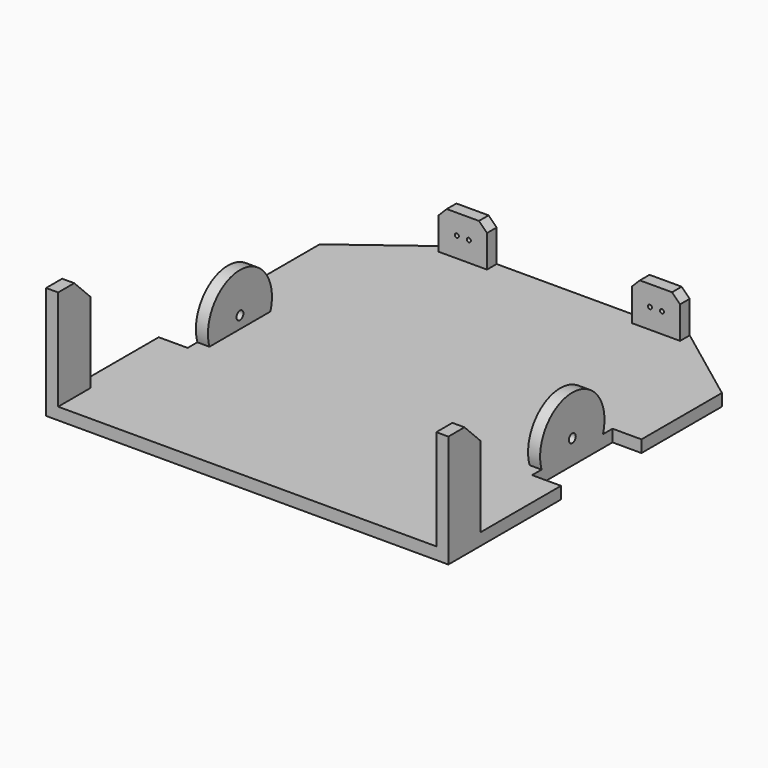
from build123d import *

# Parameters (mm, degrees)
F1_DEPTH  = 3
F2_R      = 1.075
F3_DEPTH  = 3
F4_R      = 1.075
F5_DEPTH  = 3
F6_W      = 12
F6_H      = 3
F7_DEPTH  = 10
F8_R      = 0.5
F9_DEPTH  = 3
F10_SIZE  = 2
F11_W     = 3
F11_H     = 10
F12_DEPTH = 25
F13_SIZE  = 5


# Not quite as in the source:
# - a feature names something its author has since deleted; it is built from what else it names


with BuildPart() as f1:
    # F0 (on Top) → F1 (new body)
    with BuildSketch(Plane.XY):
        Polygon((30, 56.1203770339), (-30, 56.1203770339), (-50, 41.1203770339), (-50, 16.1203770339), (-42.8093671799, 16.1203770339), (-42.8093671799, -8.8796229661), (-50, -8.8796229661), (-50, -43.8796229661), (50, -43.8796229661), (50, -8.8796229661), (42.8093671799, -8.8796229661), (42.8093671799, 16.1203770339), (50, 16.1203770339), (50, 41.1203770339), align=None)
    extrude(amount=F1_DEPTH)

    # F2 (on face) → F3 (join)
    with BuildSketch(Plane.YZ.offset(42.8093671799)):
        with BuildLine():
            Line((-5.9190149802, 3), (13.1597690481, 3))
            ThreePointArc((13.1597690481, 3), (3.6203770339, 16), (-5.9190149802, 3))
        make_face()
        with Locations((3.6203770339, 6)):
            Circle(F2_R, mode=Mode.SUBTRACT)
    extrude(amount=-F3_DEPTH)

    # F4 (on face) → F5 (join)
    with BuildSketch(Plane(origin=(-42.8093671799, 0, 0), x_dir=(0, -1, 0), z_dir=(-1, 0, 0))):
        with BuildLine():
            Line((-13.1019409746, 3), (5.8611869067, 3))
            ThreePointArc((5.8611869067, 3), (-3.6203770339, 15.9448506656), (-13.1019409746, 3))
        make_face()
        with Locations((-3.6203770339, 6)):
            Circle(F4_R, mode=Mode.SUBTRACT)
    extrude(amount=-F5_DEPTH)

    # F6 (on face) → F7 (join)
    with BuildSketch(Plane.XY.offset(3)):
        with Locations((-24, 54.6203770339)):
            Rectangle(F6_W, F6_H)
        with Locations((24, 54.6203770339)):
            Rectangle(F6_W, F6_H)
    extrude(amount=F7_DEPTH)

    # F8 (on face) → F9 (cut, through all)
    with BuildSketch(Plane(origin=(0, 56.1203770339, 0), x_dir=(-1, 0, 0), z_dir=(0, 1, 0))):
        with Locations((-25.5, 8)):
            Circle(F8_R)
        with Locations((-22.5, 8)):
            Circle(F8_R)
        with Locations((25.5, 8)):
            Circle(F8_R)
        with Locations((22.5, 8)):
            Circle(F8_R)
    extrude(amount=-F9_DEPTH, mode=Mode.SUBTRACT)

    # F10
    f10_edges = [f1.edges().sort_by_distance(p)[0] for p in [
        (18, 54.620377, 13),
        (30, 54.620377, 13),
        (-18, 54.620377, 13),
        (-30, 54.620377, 13),
    ]]
    chamfer(f10_edges, length=F10_SIZE)

    # F11 (on face) → F12 (join)
    with BuildSketch(Plane.XY.offset(3)):
        with Locations((48.5, -38.8796229661)):
            Rectangle(F11_W, F11_H)
        with Locations((-48.5, -38.8796229661)):
            Rectangle(F11_W, F11_H)
    extrude(amount=F12_DEPTH)

    # F13
    f13_edges = [f1.edges().sort_by_distance(p)[0] for p in [
        (-48.5, -33.879623, 28),
        (48.5, -33.879623, 28),
    ]]
    chamfer(f13_edges, length=F13_SIZE)


solid = f1.part
